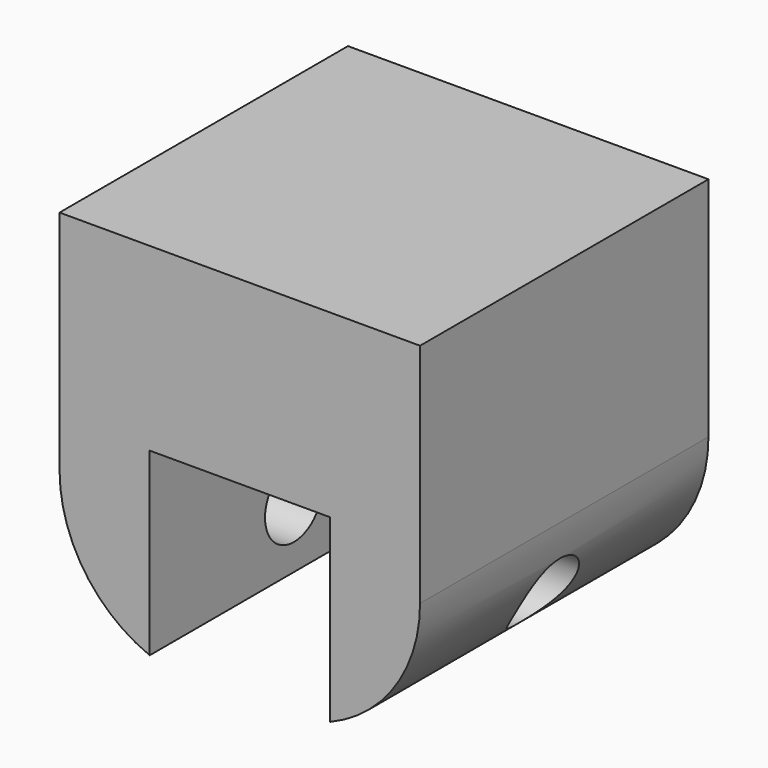
from build123d import *

# Parameters (mm, degrees)
F0_W        = 12.7
F0_H        = 12.7
F1_DEPTH    = 12.7
F2_W        = 6.35
F2_H        = 35.1087670878
F3_DEPTH    = 6.35
F4_R        = 1.27
F5_DEPTH    = 25.4
F6_T1_DEPTH = 36.2464301965


# Not quite as in the source:
# - a fillet or chamfer that OpenCascade refuses, or shapes differently, is made with other operations: its cross-section is extruded or revolved along the edge and cut away or added


with BuildPart() as f1:
    # F0 (on Top) → F1 (new body)
    with BuildSketch(Plane.XY):
        Rectangle(F0_W, F0_H)
    extrude(amount=F1_DEPTH)

    # F2 (on face) → F3 (cut)
    with BuildSketch(Plane(origin=(0, 0, 0), x_dir=(1, 0, 0), z_dir=(0, 0, -1))):
        Rectangle(F2_W, F2_H)
    extrude(amount=-F3_DEPTH, mode=Mode.SUBTRACT)

    # F4 (on face) → F5 (cut)
    with BuildSketch(Plane(origin=(-6.35, 0, 0), x_dir=(0, -1, 0), z_dir=(-1, 0, 0))):
        with Locations((0, 2.2022052582)):
            Circle(F4_R)
    extrude(amount=-F5_DEPTH, mode=Mode.SUBTRACT)

    # F6: fillet of radius 5.08 on 2 edges, made by hand

    # F6_s2 → F6_t1 (cut)
    with BuildSketch(Plane.XZ.offset(-18.1232150983)):
        with BuildLine():
            ThreePointArc((-3.175, 0), (-5.4821134838, 1.8694797079), (-6.35, 4.7092860393))
            Line((-6.35, 4.7092860393), (-6.35, 0))
            Line((-6.35, 0), (-3.175, 0))
        make_face()
        with BuildLine():
            ThreePointArc((3.175, 0), (5.4821134838, 1.8694797079), (6.35, 4.7092860393))
            Line((6.35, 4.7092860393), (6.35, 0))
            Line((6.35, 0), (3.175, 0))
        make_face()
    extrude(amount=F6_T1_DEPTH, mode=Mode.SUBTRACT)


solid = f1.part
